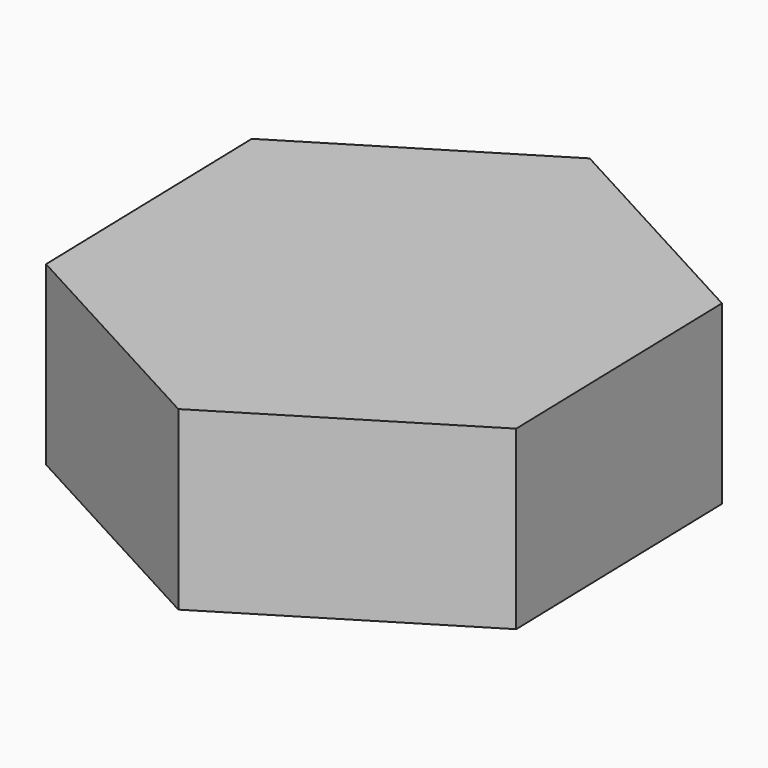
from build123d import *

# Parameters (mm, degrees)
F1_DEPTH = 25.4


# Not quite as in the source:
# - the program builds the solid bodies; features that only make, move or delete a surface that nothing else refers to are left out


with BuildPart() as f1:
    # F0 (on Top) → F1 (new body)
    with BuildSketch(Plane.XY):
        Polygon((-1.0046077546, 38.2428395196), (-33.6215744141, 18.2514039234), (-32.6169666595, -19.9914355961), (1.0046077546, -38.2428395196), (33.6215744141, -18.2514039234), (32.6169666595, 19.9914355961), align=None)
    extrude(amount=F1_DEPTH)


solid = f1.part
